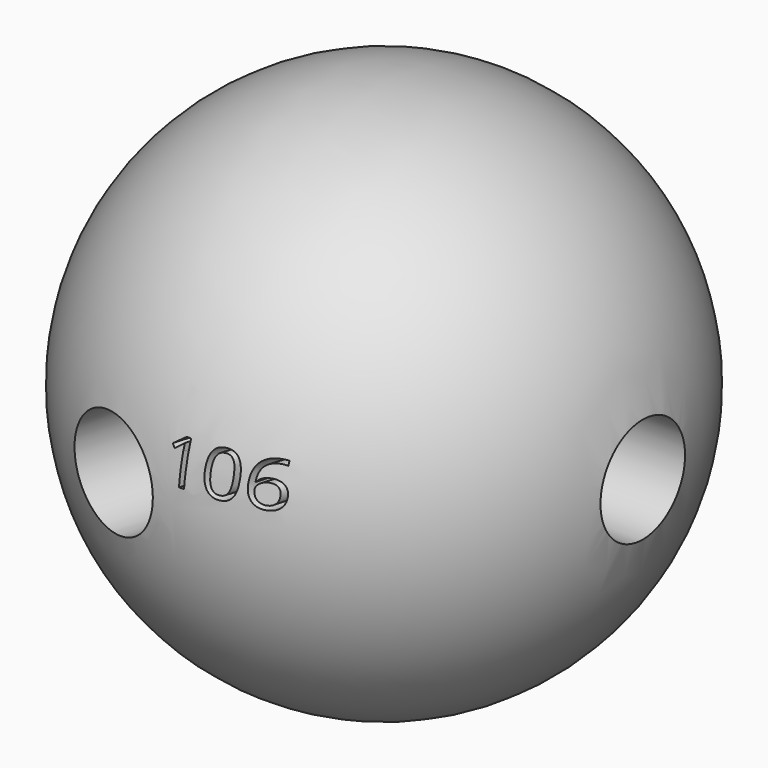
from build123d import *

# Parameters (mm, degrees)
F4_R          = 3.175
F5_DEPTH      = 25.4
F6_ANGLE      = 106
F8_ANGLE      = -90
F10_TEXT_SIZE = 3.5912789624
F11_DEPTH     = 10.6426


# Not quite as in the source:
# - Text() gives the source's letters only with a copy of the font that has no kerning and outlines rounded to 1/6400 em; it was checked with that copy


with BuildPart() as f1:
    # F0 (on Top) → F1 (revolve)
    with BuildSketch(Plane.XY):
        with BuildLine():
            Line((0, -15.875), (0, 15.875))
            ThreePointArc((0, 15.875), (-15.875, 0), (0, -15.875))
        make_face()
    revolve(axis=Axis((0, 0, 0), (0, -1, 0)))


with BuildPart() as f5:
    # F4 (on offset) → F5 (new body)
    with BuildSketch(Plane.XY.offset(6.35)):
        Circle(F4_R)
    extrude(amount=F5_DEPTH)


with BuildPart() as f6_1:
    # F6: copy of F5
    add(f5.part.rotate(Axis((37.5162102282, 0, 0), (1, 0, 0)), F6_ANGLE))


with BuildPart() as f1_1:
    add(f1.part)

    # F7: cut F6_1, F5
    add(f6_1.part, mode=Mode.SUBTRACT)
    add(f5.part, mode=Mode.SUBTRACT)


with BuildPart() as f1_2:
    # F8: moved
    add(f1_1.part.rotate(Axis((0, -28.2062906772, 0), (0, -1, 0)), F8_ANGLE))

    # F10 (on offset) → F11 (cut)
    with BuildSketch(Plane(origin=(-6.0350247781, -21.0466325802, 0), x_dir=(0.9612616959, -0.2756373558, 0), z_dir=(-0.2756373558, -0.9612616959, 0))):
        with Locations((3.724938957, 1.0774264811)):
            Text('106', F10_TEXT_SIZE, font='Open Sans', text_align=(TextAlign.LEFT, TextAlign.BOTTOM))
    extrude(amount=-F11_DEPTH, mode=Mode.SUBTRACT)


solid = f1_2.part
